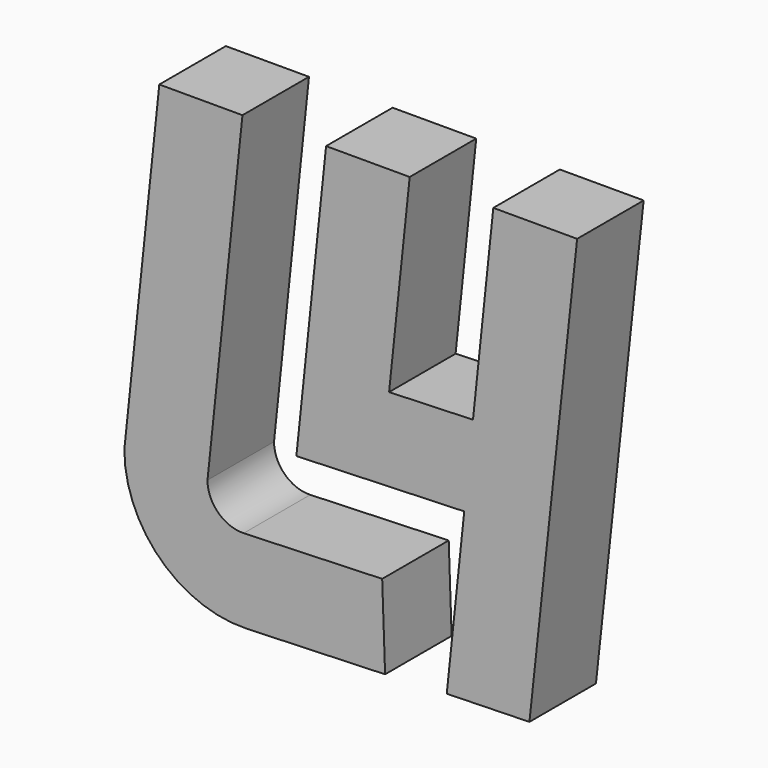
from build123d import *

# Parameters (mm, degrees)
F2_W      = 38.1
F2_H      = 38.1
F3_FACE_W = 38.1
F3_FACE_H = 38.1
F6_ANGLE  = 92
F10_DEPTH = 38.1


# Not quite as in the source:
# - a feature of the source that left no trace in its solid (it failed there, or was rolled back) is left out


with BuildPart() as f3:
    # F3: sweep along a path in F1
    with BuildLine(Plane.XZ) as f3_path:
        Line((0, 76.2), (-16.0178854545, -76.2))
    # F2 (on offset) → F3 (sweep)
    with BuildSketch(Plane.XY.offset(76.2)):
        Rectangle(F2_W, F2_H)
    sweep(path=f3_path.line)

    # F3_face (on face) → F6 (revolve)
    with BuildSketch(Plane(origin=(-16.0178854545, 0, -76.2), x_dir=(1, 0, 0), z_dir=(0, 0, -1))):
        Rectangle(F3_FACE_W, F3_FACE_H)
    revolve(axis=Axis((19.05, 0, -76.2), (0, -1, 0)), revolution_arc=F6_ANGLE)

    # F9 (on offset) → F10 (join)
    with BuildSketch(Plane.XZ.offset(-19.05)):
        with BuildLine():
            Line((19.05, 76.2), (-19.05, 76.2))
            Line((-19.05, 76.2), (-35.0678854545, -76.2))
            ThreePointArc((-35.0678854545, -76.2), (-18.5434421225, -115.1291489176), (20.938686965, -130.2849183009))
            Line((20.938686965, -130.2849183009), (84.4000044807, -128.0688002603))
            Line((84.4000044807, -128.0688002603), (83.0703336563, -89.9920097509))
            Line((83.0703336563, -89.9920097509), (19.6090161406, -92.2081277915))
            ThreePointArc((19.6090161406, -92.2081277915), (7.923041792, -87.7223025247), (3.0321145455, -76.2))
            Line((3.0321145455, -76.2), (19.05, 76.2))
        make_face()
    extrude(amount=F10_DEPTH)


with BuildPart() as f10:
    # F9 (on offset) → F10, piece 2 (new body)
    with BuildSketch(Plane.XZ.offset(-19.05)):
        Polygon((57.3598628922, 76.1999756512), (48.2847232605, -10.1442102778), (43.7549937167, -53.2417080366), (120.6569795756, -50.556231515), (112.6531418084, -126.7076610645), (150.5274446174, -125.7595791662), (172.3890340576, 76.2), (133.9795978448, 76.2000141826), (124.6786526722, -12.292567958), (86.2276597428, -13.6353062188), (95.6697283436, 76.1999756512), align=None)
    extrude(amount=F10_DEPTH)


solid = Compound([f3.part, f10.part])
